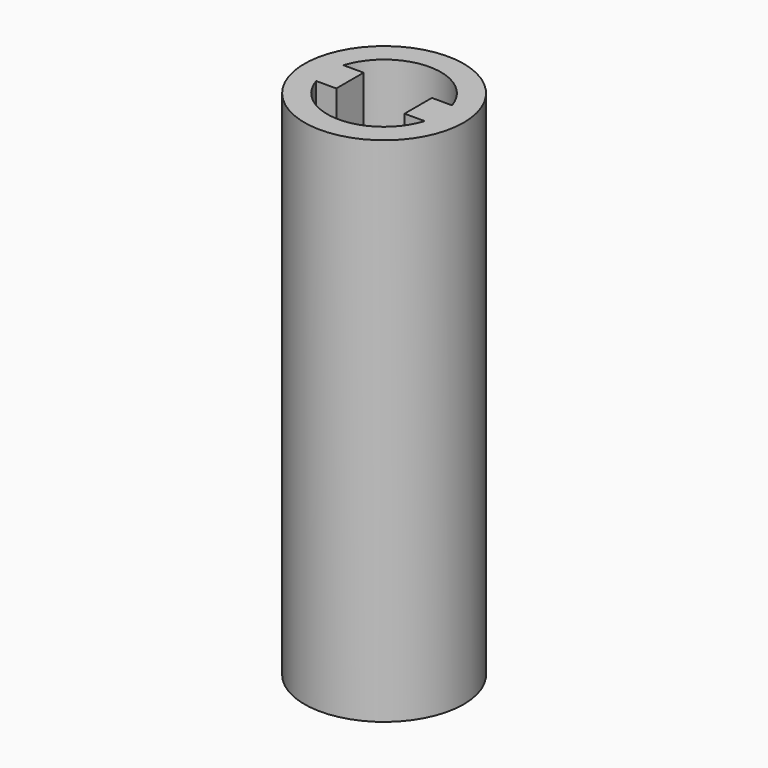
from build123d import *

# Parameters (mm, degrees)
F0_R     = 7
F1_DEPTH = 45
F3_DEPTH = 25
F4_R     = 2.55
F5_DEPTH = 10
F7_DEPTH = 4
F8_DEPTH = 10


with BuildPart() as f1:
    # F0 (on Top) → F1 (new body)
    with BuildSketch(Plane.XY):
        Circle(F0_R)
    extrude(amount=F1_DEPTH)

    # F2 (on face) → F3 (cut)
    with BuildSketch(Plane.XY.offset(45)):
        with BuildLine():
            ThreePointArc((4.7696960071, 1.5), (0, 5), (-4.7696960071, 1.5))
            Line((-4.7696960071, 1.5), (-3, 1.5))
            Line((-3, 1.5), (-3, -1.5))
            Line((-3, -1.5), (-4.7696960071, -1.5))
            ThreePointArc((-4.7696960071, -1.5), (0, -5), (4.7696960071, -1.5))
            Line((4.7696960071, -1.5), (3, -1.5))
            Line((3, -1.5), (3, 1.5))
            Line((3, 1.5), (4.7696960071, 1.5))
        make_face()
    extrude(amount=-F3_DEPTH, mode=Mode.SUBTRACT)

    # F4 (on face) → F5 (cut)
    with BuildSketch(Plane(origin=(0, 0, 0), x_dir=(1, 0, 0), z_dir=(0, 0, -1))):
        Circle(F4_R)
    extrude(amount=-F5_DEPTH, mode=Mode.SUBTRACT)

    # F6 (on face) → F7 (cut)
    with BuildSketch(Plane(origin=(0, 0, 10), x_dir=(1, 0, 0), z_dir=(0, 0, -1))):
        with BuildLine():
            Line((-1.5, 2), (-1.5, -2))
            ThreePointArc((-1.5, -2), (2.5, 0), (-1.5, 2))
        make_face()
    extrude(amount=-F7_DEPTH, mode=Mode.SUBTRACT)

    # F8 (add): a face of the model
    f8_faces = [f1.faces().sort_by_distance(p)[0] for p in [
        (-2.4778751083, 0, 10),
    ]]
    extrude(f8_faces, amount=F8_DEPTH)


solid = f1.part
